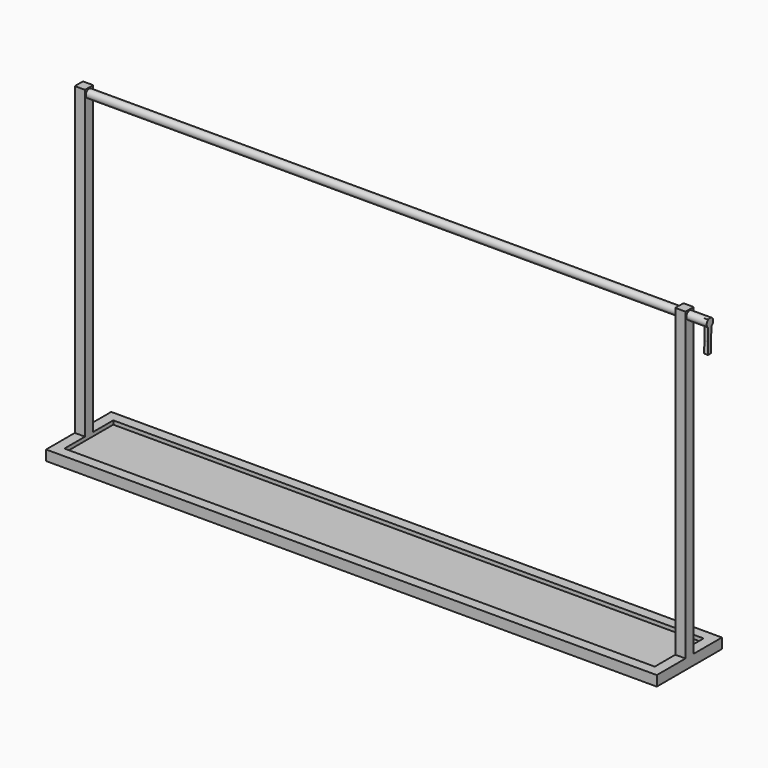
from build123d import *

# Parameters (mm, degrees)
F0_W      = 3000
F0_H      = 400
F0_W_2    = 2900
F0_H_2    = 300
F1_DEPTH  = 25
F3_DEPTH  = 1500
F4_R      = 20
F5_DEPTH  = 3064.82128
F6_R      = 20
F7_DEPTH  = 3100
F9_DEPTH  = 18.79415
F12_DEPTH = 6.35


# Not quite as in the source:
# - a feature names something its author has since deleted; it is built from what else it names
# - the program builds the solid bodies; features that only make, move or delete a surface that nothing else refers to are left out


with BuildPart() as f1:
    # F0 (on Top) → F1 (new body, symmetric)
    with BuildSketch(Plane.XY):
        Rectangle(F0_W, F0_H)
        Rectangle(F0_W_2, F0_H_2, mode=Mode.SUBTRACT)
    extrude(amount=F1_DEPTH, both=True)

    # F2 (on face) → F3 (join)
    with BuildSketch(Plane.XY.offset(25)):
        Polygon((-1500, 26.3704165816), (-1500, 0), (-1500, -23.6295834184), (-1450, -23.6295834184), (-1450, 26.3704165816), align=None)
        Polygon((1500, -23.6295834184), (1500, 0), (1500, 26.3704165816), (1450, 26.3704165816), (1450, -23.6295834184), align=None)
    extrude(amount=F3_DEPTH)

    # F4 (on face) → F5 (cut)
    with BuildSketch(Plane(origin=(-1500, 0, 0), x_dir=(0, -1, 0), z_dir=(-1, 0, 0))):
        with Locations((-1.3704165816, 1500)):
            Circle(F4_R)
    extrude(amount=-F5_DEPTH, mode=Mode.SUBTRACT)

    # F0 (on Top) → F12 (join, symmetric)
    with BuildSketch(Plane.XY):
        Rectangle(F0_W_2, F0_H_2)
    extrude(amount=F12_DEPTH, both=True)


with BuildPart() as f7:
    # F6 (on face) → F7 (new body)
    with BuildSketch(Plane(origin=(-1500, 0, 0), x_dir=(0, -1, 0), z_dir=(-1, 0, 0))):
        with Locations((-1.3704165816, 1500)):
            Circle(F6_R)
    extrude(amount=-F7_DEPTH)

    # F8 (on face) → F9 (join)
    with BuildSketch(Plane.YZ.offset(1600)):
        Polygon((-9.4648035193, 1420.9684346451), (-10.6437923387, 1364.5441532135), (7.7239090577, 1364.5441532135), (10.9214369768, 1517.5720803951), (-9.4648035193, 1517.5720803951), align=None)
    extrude(amount=-F9_DEPTH)


solid = Compound([f1.part, f7.part])
